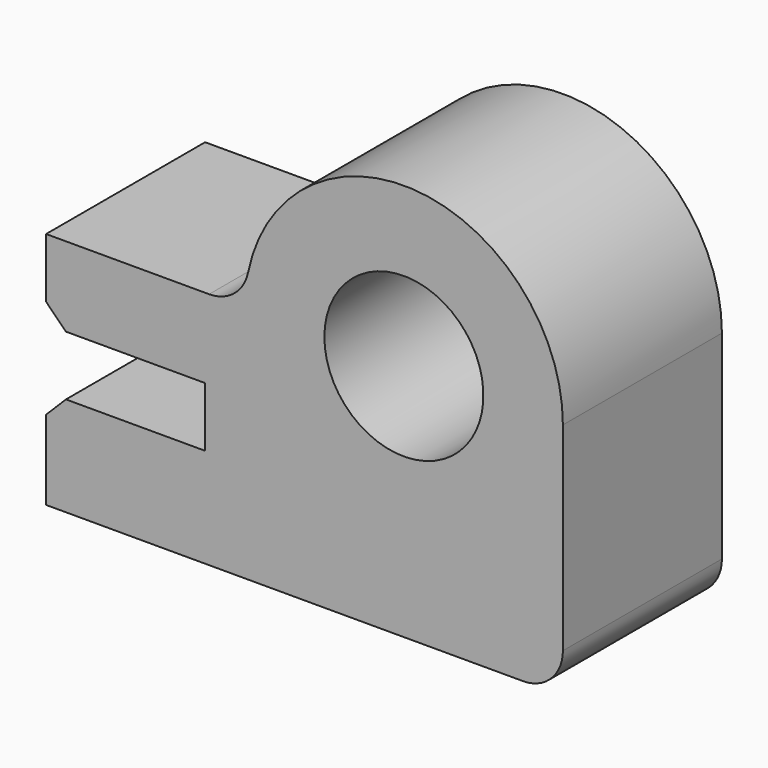
from build123d import *

# Parameters (mm, degrees)
F1_DEPTH = 50
F2_R     = 10
F3_SIZE  = 5


with BuildPart() as f1:
    # F0 (on Front) → F1 (new body)
    with BuildSketch(Plane.XZ):
        with BuildLine():
            Line((-130, 0), (0, 0))
            Line((0, 0), (0, 60))
            Line((0, 60), (-20, 60))
            ThreePointArc((-20, 60), (-40, 40), (-60, 60))
            Line((-60, 60), (-80, 60))
            Line((-80, 60), (-130, 60))
            Line((-130, 60), (-130, 40))
            Line((-130, 40), (-90, 40))
            Line((-90, 40), (-90, 25))
            Line((-90, 25), (-130, 25))
            Line((-130, 25), (-130, 0))
        make_face()
        with BuildLine():
            Line((-20, 60), (0, 60))
            ThreePointArc((0, 60), (-40, 100), (-80, 60))
            Line((-80, 60), (-60, 60))
            ThreePointArc((-60, 60), (-40, 80), (-20, 60))
        make_face()
    extrude(amount=F1_DEPTH)

    # F2
    f2_edges = [f1.edges().sort_by_distance(p)[0] for p in [
        (0, -25, 60),
        (0, -25, 0),
        (-80, -25, 60),
    ]]
    fillet(f2_edges, radius=F2_R)

    # F3
    f3_edges = [f1.edges().sort_by_distance(p)[0] for p in [
        (-130, -25, 40),
        (-130, -25, 25),
    ]]
    chamfer(f3_edges, length=F3_SIZE)


solid = f1.part
